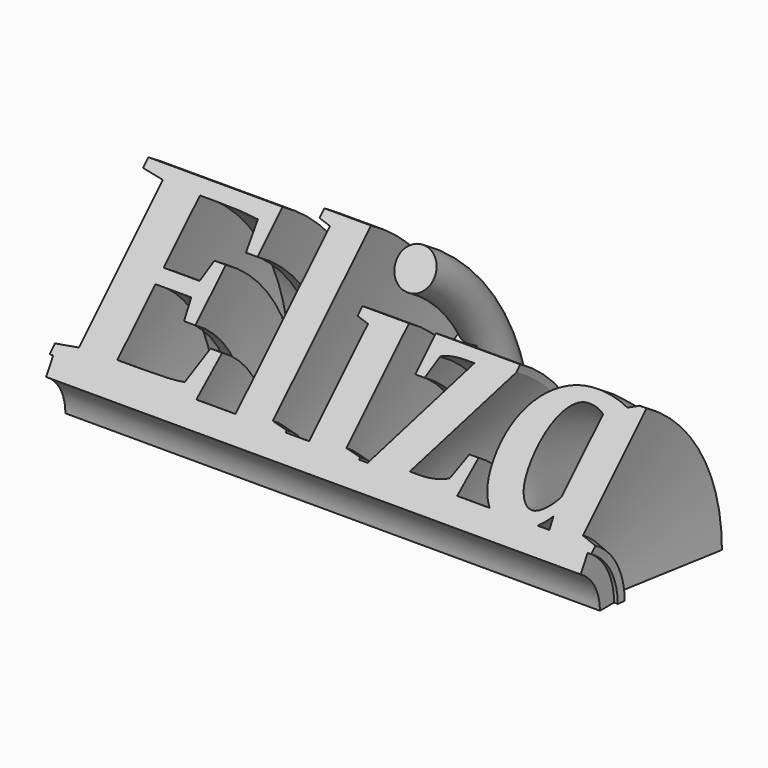
from build123d import *

# Parameters (mm, degrees)
F1_W         = 89.7409496829
F1_H         = 4.054560326
F0_TEXT_SIZE = 43.9244102583
F4_ANGLE     = 60
F2_W         = 3.5139527172
F2_H         = 8.1091211177
F5_ANGLE     = 30


# Not quite as in the source:
# - Text() gives the source's letters only with a copy of the font that has no kerning and outlines rounded to 1/6400 em; it was checked with that copy


with BuildPart() as f4:
    # F1 (on Top) + F0 (on Top) → F4 (revolve)
    with BuildSketch(Plane.XY):
        with Locations((-31.0173914768, -16.2858185358)):
            Rectangle(F1_W, F1_H)
    with BuildSketch(Plane.XY):
        with Locations((-76.1581659317, -15.3397554532)):
            Text('Eliza', F0_TEXT_SIZE, font='Tinos', font_style=FontStyle.BOLDITALIC, text_align=(TextAlign.LEFT, TextAlign.BOTTOM))
    revolve(axis=Axis((-22.6379651576, -26.4222230762, 0), (1, 0, 0)), revolution_arc=F4_ANGLE)

    # F2 (on Top) → F5 (revolve)
    with BuildSketch(Plane.XY):
        with Locations((-26.5573738143, 7.3657853063)):
            Rectangle(F2_W, F2_H)
    revolve(axis=Axis((-22.6379651576, -26.4222230762, 0), (1, 0, 0)), revolution_arc=F5_ANGLE)


solid = f4.part
